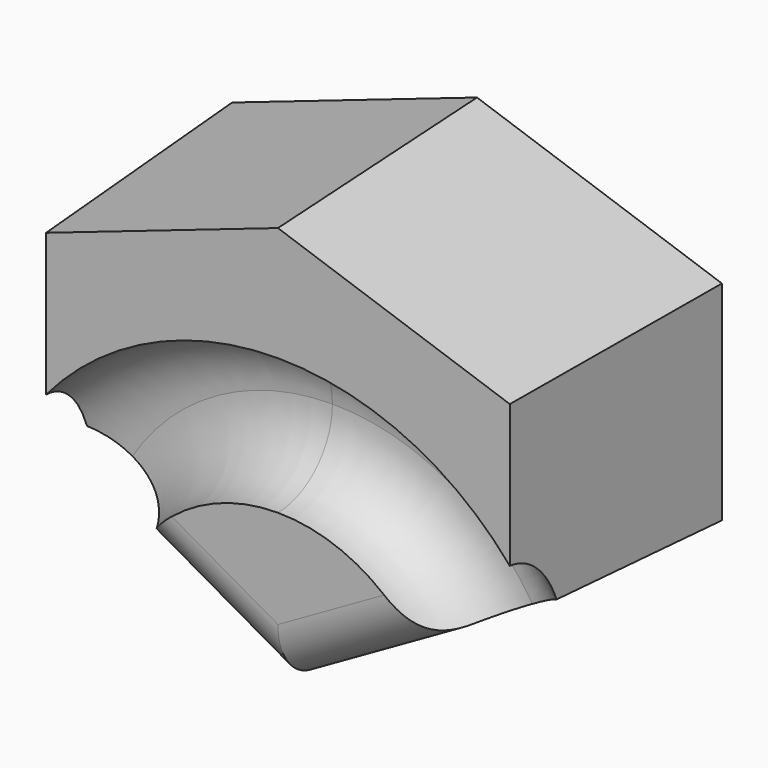
from build123d import *

# Parameters (mm, degrees)
F1_DEPTH               = 50.8
DRAFT_F1_DRAFTED_ANGLE = 3
F2_R                   = 13.8927201934
F4_R                   = 10.16
F5_T                   = -5.08


# Not quite as in the source:
# - an extrude with a draft is written as a straight extrude whose walls are then drafted


with BuildPart() as f1:
    # F0 (on Front) → F1 (new body)
    with BuildSketch(Plane.XZ):
        Polygon((50, 71.0625250938), (0, 88.2237195564), (-50, 71.0625250938), (-50, 28.4853828673), (0, 0), (50, 28.4853828673), align=None)
    extrude(amount=F1_DEPTH)

    # draft_F1_drafted
    draft_f1_drafted_walls = [f1.faces().sort_by_distance(p)[0] for p in [
        (50, -33.8666666667, 49.7739539805),
        (25, -33.8666666667, 79.6431223251),
        (-25, -33.8666666667, 79.6431223251),
        (-50, -33.8666666667, 49.7739539805),
        (-25, -33.8666666667, 14.2426914336),
        (25, -33.8666666667, 14.2426914336),
    ]]
    draft(draft_f1_drafted_walls, neutral_plane=Plane.XZ, angle=DRAFT_F1_DRAFTED_ANGLE)

    # F2 (on Right) → F3 (revolve, cut)
    with BuildSketch(Plane.YZ):
        with Locations((-50.8, 48.138115555)):
            Circle(F2_R)
    revolve(axis=Axis((0, -34.5127657056, 0), (0, -1, 0)), mode=Mode.SUBTRACT)

    # F4
    f4_edges = [f1.edges().sort_by_distance(p)[0] for p in [
        (14.173716, -50.8, 11.138928),
        (-14.173716, -50.8, 11.138928),
    ]]
    fillet(f4_edges, radius=F4_R)

    # F5
    f5_openings = [f1.faces().sort_by_distance(p)[0] for p in [
        (0, 0, 46.613583),
    ]]
    offset(amount=F5_T, openings=f5_openings)


solid = f1.part
